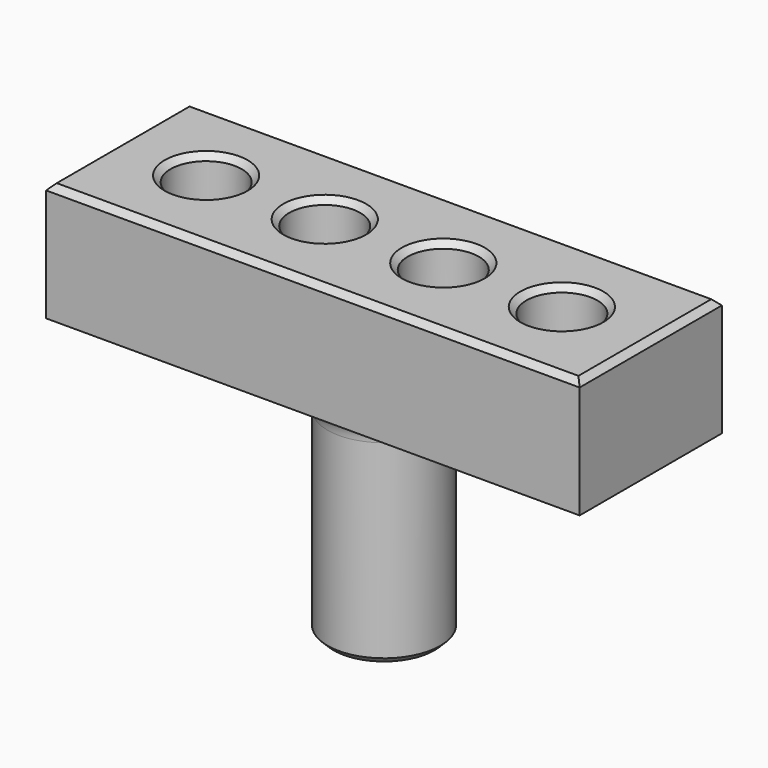
from build123d import *

# Parameters (mm, degrees)
F0_W          = 90
F0_H          = 30
F0_R          = 6
F1_DEPTH      = 20
F2_SIZE       = 1
F3_R          = 9.5
F4_DEPTH      = 5
F4_DEPTH_BACK = 38
F5_SIZE       = 1
F6_T4_ANGLE   = 359.64
F6_S5_R       = 6
F6_T6_DEPTH   = 29
F6_S7_R       = 6
F6_T8_DEPTH   = 29
F6_T12_ANGLE  = 359.64
F6_S13_R      = 6
F6_T14_DEPTH  = 29
F6_S15_R      = 6
F6_T16_DEPTH  = 29


# Not quite as in the source:
# - a fillet or chamfer that OpenCascade refuses, or shapes differently, is made with other operations: its cross-section is extruded or revolved along the edge and cut away or added


with BuildPart() as f1:
    # F0 (on Top) → F1 (new body)
    with BuildSketch(Plane.XY):
        Rectangle(F0_W, F0_H)
        with Locations((-30, 0)):
            Circle(F0_R, mode=Mode.SUBTRACT)
        with Locations((-10, 0)):
            Circle(F0_R, mode=Mode.SUBTRACT)
        with Locations((10, 0)):
            Circle(F0_R, mode=Mode.SUBTRACT)
        with Locations((30, 0)):
            Circle(F0_R, mode=Mode.SUBTRACT)
    extrude(amount=F1_DEPTH)

    # F2
    f2_edges = [f1.edges().sort_by_distance(p)[0] for p in [
        (0, 15, 20),
        (-45, 0, 20),
        (0, -15, 20),
        (45, 0, 20),
        (-36, 0, 20),
        (-16, 0, 20),
        (4, 0, 20),
        (24, 0, 20),
    ]]
    chamfer(f2_edges, length=F2_SIZE)

    # F3 (on Top) → F4 (join, two sides)
    with BuildSketch(Plane.XY) as f4_sk:
        Circle(F3_R)
    extrude(amount=F4_DEPTH)
    extrude(f4_sk.sketch, amount=-F4_DEPTH_BACK)

    # F5
    f5_edges = [f1.edges().sort_by_distance(p)[0] for p in [
        (-9.5, 0, -38),
    ]]
    chamfer(f5_edges, length=F5_SIZE)

    # F6: fillet of radius 5 on 2 edges, made by hand


with BuildPart() as f6_tool2:
    # F6_s3 → F6_t4 (revolve)
    with BuildSketch(Plane(origin=(0, 0, 0), x_dir=(0, 0, 1), z_dir=(0.9999950652, 0.0031415875, 0))):
        with BuildLine():
            ThreePointArc((-5, -9.5), (-1.4644660941, -10.9644660941), (0, -14.5))
            Line((0, -14.5), (0, -9.5))
            Line((0, -9.5), (-5, -9.5))
        make_face()
    revolve(axis=Axis((0, 0, 0), (0, 0, 1)), revolution_arc=F6_T4_ANGLE)

    # F6_s5 → F6_t6 (cut, symmetric)
    with BuildSketch(Plane.XY.offset(-2.5)):
        with Locations((10, 0)):
            Circle(F6_S5_R)
    extrude(amount=F6_T6_DEPTH, both=True, mode=Mode.SUBTRACT)

    # F6_s7 → F6_t8 (cut, symmetric)
    with BuildSketch(Plane.XY.offset(-2.5)):
        with Locations((-10, 0)):
            Circle(F6_S7_R)
    extrude(amount=F6_T8_DEPTH, both=True, mode=Mode.SUBTRACT)


with BuildPart() as f1_1:
    add(f1.part)

    # F6_t1: union F6_tool2
    add(f6_tool2.part)


with BuildPart() as f6_tool10:
    # F6_s11 → F6_t12 (revolve)
    with BuildSketch(Plane(origin=(0, 0, 0), x_dir=(0, 0, 1), z_dir=(-0.9999950652, -0.0031415875, 0))):
        with BuildLine():
            ThreePointArc((-5, -9.5), (-1.4644660941, -10.9644660941), (0, -14.5))
            Line((0, -14.5), (0, -9.5))
            Line((0, -9.5), (-5, -9.5))
        make_face()
    revolve(axis=Axis((0, 0, 0), (0, 0, 1)), revolution_arc=F6_T12_ANGLE)

    # F6_s13 → F6_t14 (cut, symmetric)
    with BuildSketch(Plane.XY.offset(-2.5)):
        with Locations((10, 0)):
            Circle(F6_S13_R)
    extrude(amount=F6_T14_DEPTH, both=True, mode=Mode.SUBTRACT)

    # F6_s15 → F6_t16 (cut, symmetric)
    with BuildSketch(Plane.XY.offset(-2.5)):
        with Locations((-10, 0)):
            Circle(F6_S15_R)
    extrude(amount=F6_T16_DEPTH, both=True, mode=Mode.SUBTRACT)


with BuildPart() as f1_2:
    add(f1_1.part)

    # F6_t9: union F6_tool10
    add(f6_tool10.part)


solid = f1_2.part
